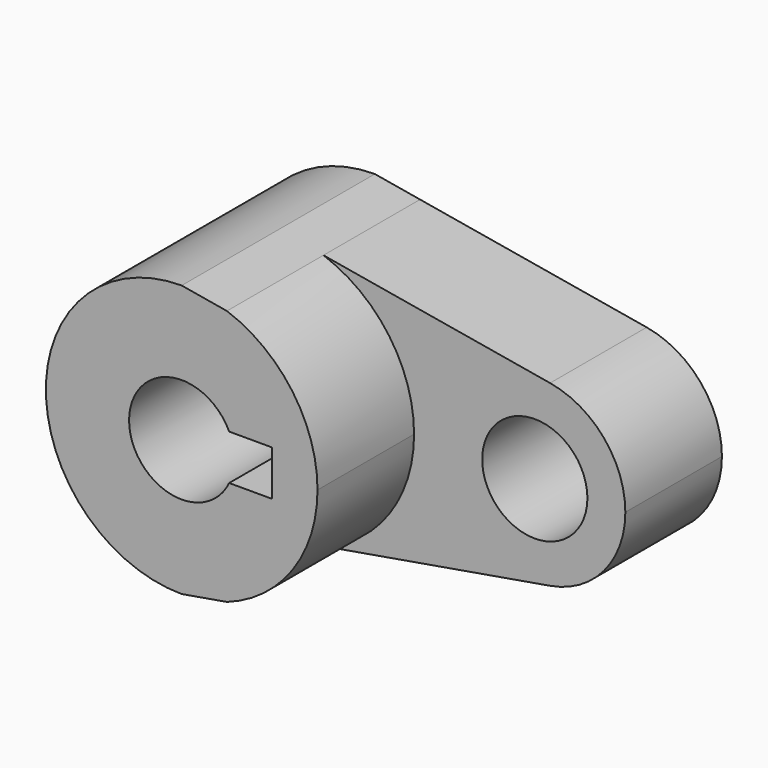
from build123d import *

# Parameters (mm, degrees)
F0_R     = 11.06846298
F1_DEPTH = 25.4
F2_DEPTH = 50.8


with BuildPart() as f1:
    # F0 (on Front) → F1 (new body)
    with BuildSketch(Plane.XZ):
        with BuildLine():
            Line((9.5121844836, 26.9452959039), (0, 28.575))
            ThreePointArc((0, 28.575), (-28.575, 0), (0, -28.575))
            Line((0, -28.575), (9.5121844836, -26.9452959039))
            ThreePointArc((9.5121844836, -26.9452959039), (23.3274655355, -16.5033322905), (28.575, 0))
            ThreePointArc((28.575, 0), (23.3274655355, 16.5033322905), (9.5121844836, 26.9452959039))
        make_face()
        with BuildLine():
            ThreePointArc((-9.9914696861, 4.7625), (0, 11.06846298), (9.9914696861, 4.7625))
            Line((9.9914696861, 4.7625), (19.05, 4.7625))
            Line((19.05, 4.7625), (19.05, -4.7625))
            Line((19.05, -4.7625), (9.9914696861, -4.7625))
            ThreePointArc((9.9914696861, -4.7625), (0, -11.06846298), (-9.9914696861, -4.7625))
            Line((-9.9914696861, -4.7625), (-19.05, -4.7625))
            Line((-19.05, -4.7625), (-19.05, 4.7625))
            Line((-19.05, 4.7625), (-9.9914696861, 4.7625))
        make_face(mode=Mode.SUBTRACT)
        with BuildLine():
            Line((57.1919272622, 18.7764181619), (9.5121844836, 26.9452959039))
            ThreePointArc((9.5121844836, 26.9452959039), (23.3274655355, 16.5033322905), (28.575, 0))
            ThreePointArc((28.575, 0), (23.3274655355, -16.5033322905), (9.5121844836, -26.9452959039))
            Line((9.5121844836, -26.9452959039), (57.1919272622, -18.7764181619))
            ThreePointArc((57.1919272622, -18.7764181619), (34.925, 0), (57.1919272622, 18.7764181619))
        make_face()
        with BuildLine():
            ThreePointArc((73.025, 0), (68.5383952831, 12.2804730295), (57.1919272622, 18.7764181619))
            ThreePointArc((57.1919272622, 18.7764181619), (34.925, 0), (57.1919272622, -18.7764181619))
            ThreePointArc((57.1919272622, -18.7764181619), (68.5383952831, -12.2804730295), (73.025, 0))
        make_face()
        with Locations((53.975, 0)):
            Circle(F0_R, mode=Mode.SUBTRACT)
        with BuildLine():
            ThreePointArc((-9.9914696861, -4.7625), (-11.06846298, 0), (-9.9914696861, 4.7625))
            Line((-9.9914696861, 4.7625), (-19.05, 4.7625))
            Line((-19.05, 4.7625), (-19.05, -4.7625))
            Line((-19.05, -4.7625), (-9.9914696861, -4.7625))
        make_face()
    extrude(amount=F1_DEPTH)

    # F0 (on Front) → F2 (join)
    with BuildSketch(Plane.XZ):
        with BuildLine():
            Line((9.5121844836, 26.9452959039), (0, 28.575))
            ThreePointArc((0, 28.575), (-28.575, 0), (0, -28.575))
            Line((0, -28.575), (9.5121844836, -26.9452959039))
            ThreePointArc((9.5121844836, -26.9452959039), (23.3274655355, -16.5033322905), (28.575, 0))
            ThreePointArc((28.575, 0), (23.3274655355, 16.5033322905), (9.5121844836, 26.9452959039))
        make_face()
        with BuildLine():
            ThreePointArc((-9.9914696861, 4.7625), (0, 11.06846298), (9.9914696861, 4.7625))
            Line((9.9914696861, 4.7625), (19.05, 4.7625))
            Line((19.05, 4.7625), (19.05, -4.7625))
            Line((19.05, -4.7625), (9.9914696861, -4.7625))
            ThreePointArc((9.9914696861, -4.7625), (0, -11.06846298), (-9.9914696861, -4.7625))
            Line((-9.9914696861, -4.7625), (-19.05, -4.7625))
            Line((-19.05, -4.7625), (-19.05, 4.7625))
            Line((-19.05, 4.7625), (-9.9914696861, 4.7625))
        make_face(mode=Mode.SUBTRACT)
        with BuildLine():
            ThreePointArc((-9.9914696861, -4.7625), (-11.06846298, 0), (-9.9914696861, 4.7625))
            Line((-9.9914696861, 4.7625), (-19.05, 4.7625))
            Line((-19.05, 4.7625), (-19.05, -4.7625))
            Line((-19.05, -4.7625), (-9.9914696861, -4.7625))
        make_face()
    extrude(amount=F2_DEPTH)


solid = f1.part
